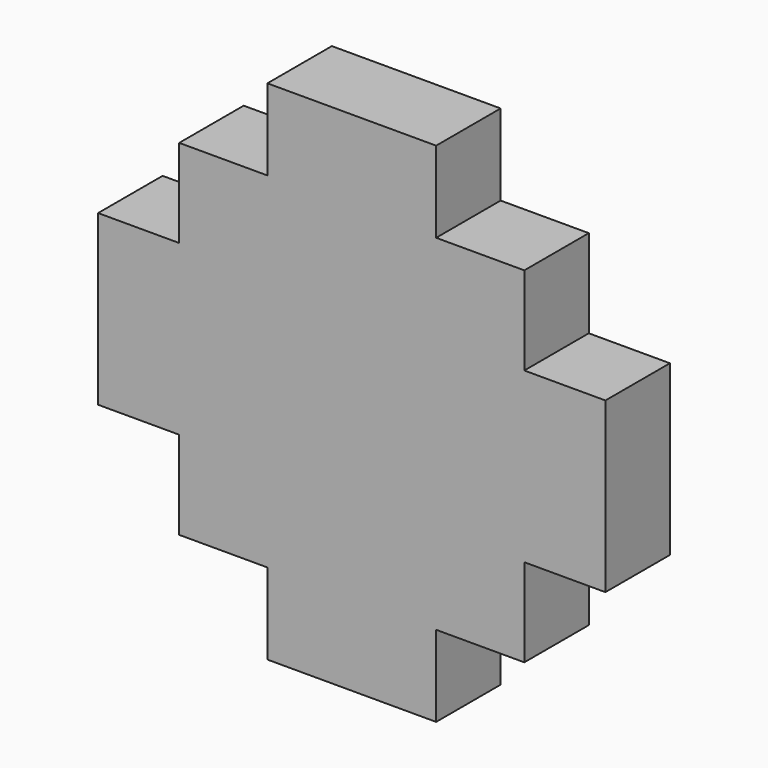
from build123d import *

# Parameters (mm, degrees)
F1_DEPTH = 2.032
F2_DEPTH = 1


# Not quite as in the source:
# - a feature names something its author has since deleted; it is built from what else it names


with BuildPart() as f1:
    # F0 (on Front) → F1 (new body)
    with BuildSketch(Plane.XZ):
        Polygon((-15.2212520439, 36.2265945869), (-17.3485020439, 36.2265945869), (-19.4757520439, 36.2265945869), (-19.4757520439, 34.1818945869), (-21.6982520439, 34.1818945869), (-21.6982520439, 31.9593945869), (-23.7429520439, 31.9593945869), (-23.7429520439, 29.8321445869), (-23.7429520439, 27.7048945869), (-21.6982520439, 27.7048945869), (-21.6982520439, 25.4823945869), (-19.4757520439, 25.4823945869), (-19.4757520439, 23.4376945869), (-17.3485020439, 23.4376945869), (-15.2212520439, 23.4376945869), (-15.2212520439, 25.4823945869), (-12.9987520439, 25.4823945869), (-12.9987520439, 27.7048945869), (-10.9540520439, 27.7048945869), (-10.9540520439, 29.8321445869), (-10.9540520439, 31.9593945869), (-12.9987520439, 31.9593945869), (-12.9987520439, 34.1818945869), (-15.2212520439, 34.1818945869), align=None)
        Polygon((-20.2887904064, 26.8476658233), (-17.9100000431, 32.8906836652), (-17.3217338641, 32.8878096037), (-14.9560986218, 26.8476658233), (-15.6798228753, 26.8476658233), (-16.4316139315, 28.7639858865), (-18.8453636264, 28.7639858865), (-19.5791117047, 26.8476658233), align=None, mode=Mode.SUBTRACT)
        Polygon((-17.3217338641, 32.8878096037), (-17.9100000431, 32.8906836652), (-20.2887904064, 26.8476658233), (-19.5791117047, 26.8476658233), (-18.8453636264, 28.7639858865), (-16.4316139315, 28.7639858865), (-15.6798228753, 26.8476658233), (-14.9560986218, 26.8476658233), align=None)
        Polygon((-18.5900452678, 29.3939520338), (-17.6306684633, 32.1173264378), (-16.6415135508, 29.3939520338), align=None, mode=Mode.SUBTRACT)
        Polygon((-16.6415135508, 29.3939520338), (-17.6306684633, 32.1173264378), (-18.5900452678, 29.3939520338), align=None)
    extrude(amount=F1_DEPTH)

    # F0 (on Front) → F2 (cut)
    with BuildSketch(Plane.XZ):
        Polygon((-17.3217338641, 32.8878096037), (-17.9100000431, 32.8906836652), (-20.2887904064, 26.8476658233), (-19.5791117047, 26.8476658233), (-18.8453636264, 28.7639858865), (-16.4316139315, 28.7639858865), (-15.6798228753, 26.8476658233), (-14.9560986218, 26.8476658233), align=None)
        Polygon((-18.5900452678, 29.3939520338), (-17.6306684633, 32.1173264378), (-16.6415135508, 29.3939520338), align=None, mode=Mode.SUBTRACT)
    extrude(amount=F2_DEPTH, mode=Mode.SUBTRACT)


solid = f1.part
